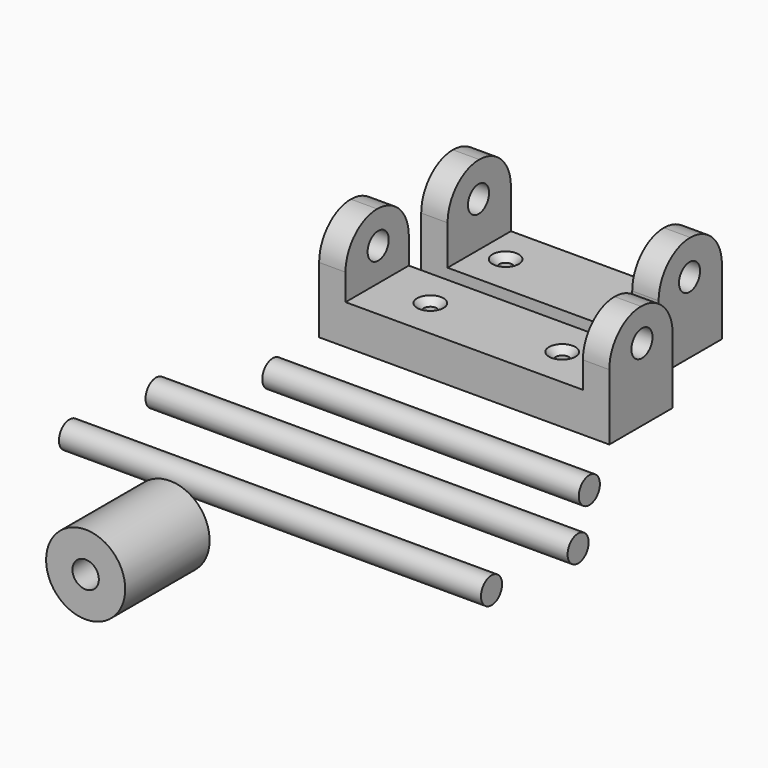
from build123d import *

# Parameters (mm, degrees)
F0_W            = 139.7
F0_H            = 38.1
F1_DEPTH        = 50.8
F2_W            = 114.3
F2_H            = 38.1
F3_DEPTH        = 31.75
F5_D            = 12.7
F7_D            = 6.35
F7_CSINK_D      = 12.7
F7_CSINK_ANGLE  = 90
F8_D            = 6.35
F8_CSINK_D      = 12.7
F8_CSINK_ANGLE  = 90
F9_W            = 114.3
F9_H            = 38.1
F10_DEPTH       = 50.8
F11_W           = 88.9
F11_H           = 38.1
F12_DEPTH       = 38.1
F14_D           = 12.7
F16_D           = 6.35
F16_CSINK_D     = 12.7
F16_CSINK_ANGLE = 90
F17_W           = 152.4
F17_H           = 6.35
F19_R           = 19.04999
F19_2_R         = 19.04999
F20_W           = 203.2
F20_H           = 6.35
F22_W           = 203.2
F22_H           = 6.35
F24_W           = 19.05
F24_H           = 50.8
F27_D           = 6.35
F27_DEPTH       = 19.051
F28_D           = 12.7


# Not quite as in the source:
# - a fillet or chamfer is up to 0.001 mm smaller than in the source, because OpenCascade refuses the exact size


with BuildPart() as f1:
    # F0 (on Top) → F1 (new body)
    with BuildSketch(Plane.XY):
        with Locations((69.85, 19.05)):
            Rectangle(F0_W, F0_H)
    extrude(amount=F1_DEPTH)

    # F2 (on face) → F3 (cut)
    with BuildSketch(Plane.XY.offset(50.8)):
        with Locations((69.85, 19.05)):
            Rectangle(F2_W, F2_H)
    extrude(amount=-F3_DEPTH, mode=Mode.SUBTRACT)

    # F5 (through all)
    with Locations(Plane(origin=(0, 0, 0), x_dir=(0, 1, 0), z_dir=(-1, 0, 0))):
        with Locations((19.6577664465, -34.9528230727)):
            Hole(F5_D / 2)

    # F7 (through all)
    with Locations(Plane.XY.offset(19.05)):
        with Locations((38.1, 19.2937536606)):
            CounterSinkHole(F7_D / 2, F7_CSINK_D / 2, counter_sink_angle=F7_CSINK_ANGLE)

    # F8 (through all)
    with Locations(Plane.XY.offset(19.05)):
        with Locations((101.6, 19.2937536606)):
            CounterSinkHole(F8_D / 2, F8_CSINK_D / 2, counter_sink_angle=F8_CSINK_ANGLE)

    # F19#2 (radius 19.05 in the source; OpenCascade refuses exactly that, so slightly less here)
    f19_2_edges = [f1.edges().sort_by_distance(p)[0] for p in [
        (6.35, 38.1, 50.8),
        (6.35, 0, 50.8),
        (133.35, 38.1, 50.8),
        (133.35, 0, 50.8),
    ]]
    fillet(f19_2_edges, radius=F19_2_R)


with BuildPart() as f10:
    # F9 (on Top) → F10 (new body)
    with BuildSketch(Plane.XY):
        with Locations((61.9886387933, 74.4279935342)):
            Rectangle(F9_W, F9_H)
    extrude(amount=F10_DEPTH)

    # F11 (on face) → F12 (cut)
    with BuildSketch(Plane.XY.offset(50.8)):
        with Locations((61.9886387933, 74.4279935342)):
            Rectangle(F11_W, F11_H)
    extrude(amount=-F12_DEPTH, mode=Mode.SUBTRACT)

    # F14 (through all)
    with Locations(Plane(origin=(0, 0, 0), x_dir=(0, 1, 0), z_dir=(-1, 0, 0))):
        with Locations((73.9847123623, -34.2443138361)):
            Hole(F14_D / 2)

    # F16 (through all)
    with Locations(Plane.XY.offset(12.7)):
        with Locations((30.2386387933, 74.4279935342), (93.7386387933, 73.8603323698)):
            CounterSinkHole(F16_D / 2, F16_CSINK_D / 2, counter_sink_angle=F16_CSINK_ANGLE)

    # F19 (radius 19.05 in the source; OpenCascade refuses exactly that, so slightly less here)
    f19_edges = [f10.edges().sort_by_distance(p)[0] for p in [
        (11.188639, 93.477994, 50.8),
        (11.188639, 55.377994, 50.8),
        (112.788639, 55.377994, 50.8),
        (112.788639, 93.477994, 50.8),
    ]]
    fillet(f19_edges, radius=F19_R)


with BuildPart() as f18:
    # F17 (on Top) → F18 (revolve)
    with BuildSketch(Plane.XY):
        with Locations((80.8163173497, -30.4894949675)):
            Rectangle(F17_W, F17_H)
    revolve(axis=Axis((80.8163173497, -33.6644949675, 0), (1, 0, 0)))


with BuildPart() as f21:
    # F20 (on Top) → F21 (revolve)
    with BuildSketch(Plane.XY):
        with Locations((81.7854143679, -70.1896044196)):
            Rectangle(F20_W, F20_H)
    revolve(axis=Axis((81.7854143679, -73.3646044196, 0), (1, 0, 0)))


with BuildPart() as f23:
    # F22 (on Top) → F23 (revolve)
    with BuildSketch(Plane.XY):
        with Locations((77.6535756886, -117.141823427)):
            Rectangle(F22_W, F22_H)
    revolve(axis=Axis((77.6535756886, -120.316823427, 0), (1, 0, 0)))


with BuildPart() as f25:
    # F24 (on Top) → F25 (revolve)
    with BuildSketch(Plane.XY):
        with Locations((42.55234483, -180.2226006985)):
            Rectangle(F24_W, F24_H)
    revolve(axis=Axis((52.07734483, -180.2226006985, 0), (0, -1, 0)))

    # F27 (through all, one way)
    with BuildSketch(Plane.XY):
        with Locations((52.07734483, -181.2174618244)):
            Circle(F27_D / 2)
    extrude(amount=-F27_DEPTH, mode=Mode.SUBTRACT)

    # F28 (through all)
    with Locations(Plane.XZ.offset(205.6226006985)):
        with Locations((52.07734483, 0)):
            Hole(F28_D / 2)


solid = Compound([f1.part, f10.part, f18.part, f21.part, f23.part, f25.part])
